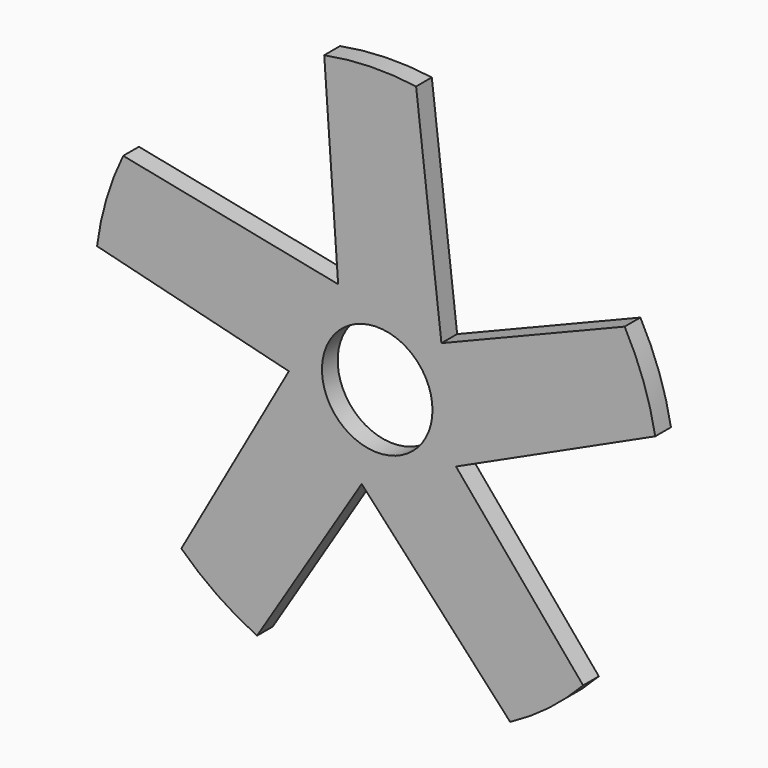
from build123d import *

# Parameters (mm, degrees)
F0_R            = 115
F0_R_2          = 22.5
F1_DEPTH        = 8
F3_DEPTH        = 25
F3_COPIES_COUNT = 5


# Not quite as in the source:
# - a pattern or mirror of a feature is missing from the dataset's text; its kind, count and spacing are read off the source's solid


with BuildPart() as f1:
    # F0 (on Front) → F1 (new body)
    with BuildSketch(Plane.XZ):
        Circle(F0_R)
        Circle(F0_R_2, mode=Mode.SUBTRACT)
    extrude(amount=F1_DEPTH)

    # F2 (on face) → F3 (cut)
    with BuildSketch(Plane.XZ.offset(8)):
        Polygon((100.7627065135, 144.0385852402), (15.8349641698, 113.9045824791), (26.1514205486, 25.2313297242), (100.7627065135, 55.4245160203), align=None)
    f3 = extrude(amount=-F3_DEPTH, mode=Mode.SUBTRACT)

    # F3_copies: F3 ×5 about axis
    f3_copies_axis = Axis((0, 0, 0), (0, 1, 0))
    for i in range(1, F3_COPIES_COUNT):
        add(f3.rotate(f3_copies_axis, i * 360 / F3_COPIES_COUNT), mode=Mode.SUBTRACT)


solid = f1.part
